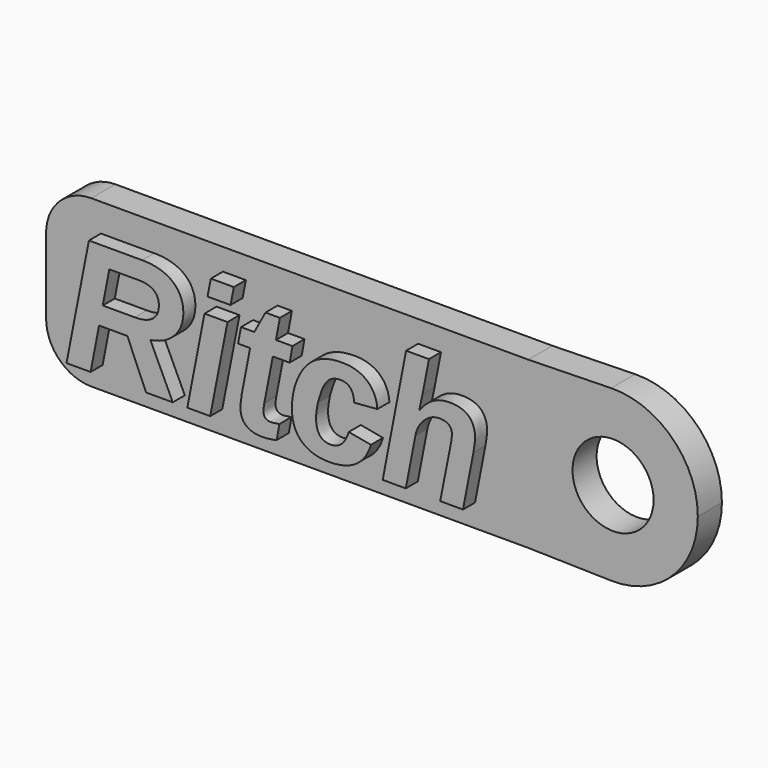
from build123d import *

# Parameters (mm, degrees)
F0_TEXT_SIZE = 11.1111111111
F1_DEPTH     = 1
F2_R         = 2.69
F3_DEPTH     = 2
F4_R         = 3


# Not quite as in the source:
# - Text() gives the source's letters only with a copy of the font that has no kerning and outlines rounded to 1/6400 em; it was checked with that copy


with BuildPart() as f1:
    # F0 (on Front) → F1 (new body)
    with BuildSketch(Plane.XZ):
        with Locations((-14.0407986111, -8)):
            Text('Ritch', F0_TEXT_SIZE, font='Arimo', font_style=FontStyle.BOLDITALIC, text_align=(TextAlign.LEFT, TextAlign.BOTTOM))
    extrude(amount=F1_DEPTH)


with BuildPart() as f3:
    # F2 (on Front) → F3 (new body)
    with BuildSketch(Plane.XZ):
        with BuildLine():
            Line((-16, -9.5), (16, -9.5))
            Line((16, -9.5), (21.4986114618, -9.6235799041))
            ThreePointArc((21.4986114618, -9.6235799041), (16, -4), (21.4986114618, 1.6235799041))
            Line((21.4986114618, 1.6235799041), (16, 1.5))
            Line((16, 1.5), (-16, 1.5))
            Line((-16, 1.5), (-16, -9.5))
        make_face()
        with BuildLine():
            ThreePointArc((21.4986114618, 1.6235799041), (16, -4), (21.4986114618, -9.6235799041))
            ThreePointArc((21.4986114618, -9.6235799041), (25.5575366796, -8.0219125132), (27.25, -4))
            ThreePointArc((27.25, -4), (25.5575366796, 0.0219125132), (21.4986114618, 1.6235799041))
        make_face()
        with Locations((21.625, -4)):
            Circle(F2_R, mode=Mode.SUBTRACT)
    extrude(amount=-F3_DEPTH)

    # F4
    f4_edges = [f3.edges().sort_by_distance(p)[0] for p in [
        (-16, 1, 1.5),
        (-16, 1, -9.5),
        (16, 1, -9.5),
        (16, 1, 1.5),
    ]]
    fillet(f4_edges, radius=F4_R)


solid = Compound([f1.part, f3.part])
